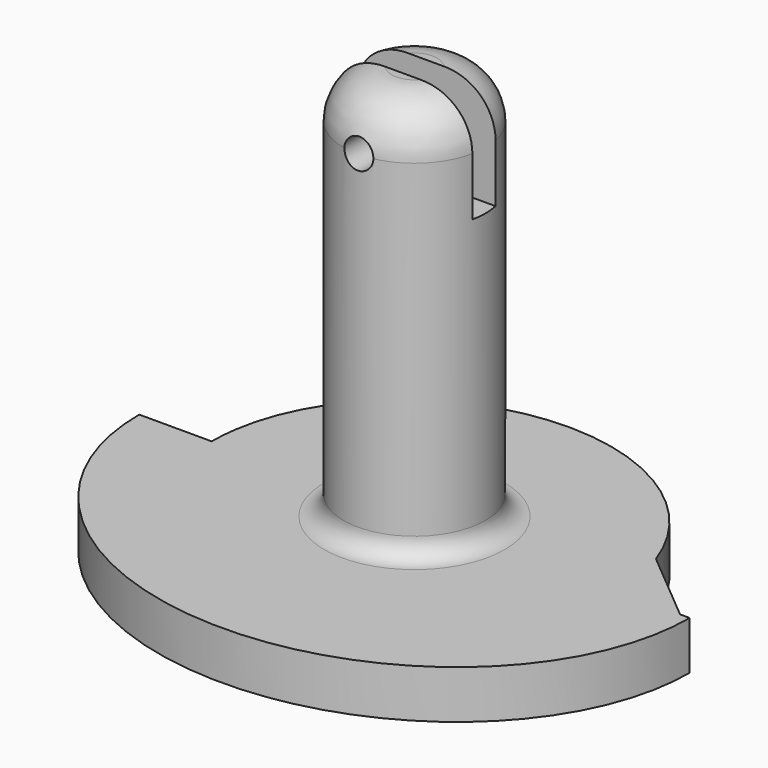
from build123d import *

# Parameters (mm, degrees)
F0_R          = 9
F0_R_2        = 7.35
F1_DEPTH      = 5
F2_DEPTH      = 46
F3_W          = 14.3906219463
F3_H          = 3
F4_DEPTH      = 11
F5_R          = 5
F6_R          = 1.5
F7_DEPTH      = 25
F7_DEPTH_BACK = 25
F8_R          = 2


# Not quite as in the source:
# - a feature names something its author has since deleted; it is built from what else it names


with BuildPart() as f1:
    # F0 (on Top) → F1 (new body)
    with BuildSketch(Plane.XY):
        with BuildLine():
            add(Edge.make_bspline(
                [(19.9054758651, 6.3725624005), (14.2198809993, 22.4810875589), (-3.3900595004, 19.737678704), (-21, 16.994269849), (-21, 0)],
                knots=[3.4658744739, 3.4658744739, 3.4658744739, 4.8745298905, 4.8745298905, 6.2831853072, 6.2831853072, 6.2831853072], degree=2, weights=[1, 0.7620470474, 1, 0.7620470474, 1]))
            add(Edge.make_bspline(
                [(-21, 0), (-21, -20), (0, -20), (21, -20), (21, 0)],
                knots=[0, 0, 0, 1.5707963268, 1.5707963268, 3.1415926536, 3.1415926536, 3.1415926536], degree=2, weights=[1, 0.7071067812, 1, 0.7071067812, 1]))
            add(Edge.make_bspline(
                [(21, 0), (21, 3.2715377973), (19.9054758651, 6.3725624005)],
                knots=[3.1415926536, 3.1415926536, 3.1415926536, 3.4658744739, 3.4658744739, 3.4658744739], degree=2, weights=[1, 0.9868839352, 1]))
        make_face()
        Circle(F0_R, mode=Mode.SUBTRACT)
        with BuildLine():
            add(Edge.make_bspline(
                [(-28.5, 0), (-28.5, -25), (0, -25), (28.5, -25), (28.5, 0)],
                knots=[3.1415926536, 3.1415926536, 3.1415926536, 4.7123889804, 4.7123889804, 6.2831853072, 6.2831853072, 6.2831853072], degree=2, weights=[1, 0.7071067812, 1, 0.7071067812, 1]))
            Line((28.5, 0), (27.5, 0))
            Line((27.5, 0), (21, 0))
            add(Edge.make_bspline(
                [(-21, 0), (-21, -20), (0, -20), (21, -20), (21, 0)],
                knots=[0, 0, 0, 1.5707963268, 1.5707963268, 3.1415926536, 3.1415926536, 3.1415926536], degree=2, weights=[1, 0.7071067812, 1, 0.7071067812, 1]))
            Line((-21, 0), (-28.5, 0))
        make_face()
        Circle(F0_R)
        Circle(F0_R_2, mode=Mode.SUBTRACT)
        Circle(F0_R_2)
        with BuildLine():
            Line((21, 0), (27.5, 0))
            Line((27.5, 0), (19.9054758651, 6.3725624005))
            add(Edge.make_bspline(
                [(21, 0), (21, 3.2715377973), (19.9054758651, 6.3725624005)],
                knots=[3.1415926536, 3.1415926536, 3.1415926536, 3.4658744739, 3.4658744739, 3.4658744739], degree=2, weights=[1, 0.9868839352, 1]))
        make_face()
    extrude(amount=F1_DEPTH)

    # F0 (on Top) → F2 (join)
    with BuildSketch(Plane.XY):
        Circle(F0_R_2)
    extrude(amount=F2_DEPTH)

    # F3 (on face) → F4 (cut)
    with BuildSketch(Plane.XY.offset(46)):
        Rectangle(F3_W, F3_H)
        with BuildLine():
            Line((-7.1953109731, -1.5), (-7.1953109731, 1.5))
            ThreePointArc((-7.1953109731, 1.5), (-7.35, 0), (-7.1953109731, -1.5))
        make_face()
        with BuildLine():
            ThreePointArc((7.35, 0), (7.3112254668, 0.7539775685), (7.1953109731, 1.5))
            Line((7.1953109731, 1.5), (7.1953109731, -1.5))
            ThreePointArc((7.1953109731, -1.5), (7.3112254668, -0.7539775685), (7.35, 0))
        make_face()
    extrude(amount=-F4_DEPTH, mode=Mode.SUBTRACT)

    # F5
    f5_edges = [f1.edges().sort_by_distance(p)[0] for p in [
        (0, -7.35, 46),
        (0, 7.35, 46),
    ]]
    fillet(f5_edges, radius=F5_R)

    # F6 (on face) → F7 (cut, two sides)
    with BuildSketch(Plane.XZ.offset(-1.5)) as f7_sk:
        with Locations((0, 41)):
            Circle(F6_R)
    extrude(amount=-F7_DEPTH, mode=Mode.SUBTRACT)
    extrude(f7_sk.sketch, amount=F7_DEPTH_BACK, mode=Mode.SUBTRACT)

    # F8
    f8_edges = [f1.edges().sort_by_distance(p)[0] for p in [
        (-7.35, 0, 5),
    ]]
    fillet(f8_edges, radius=F8_R)


solid = f1.part
